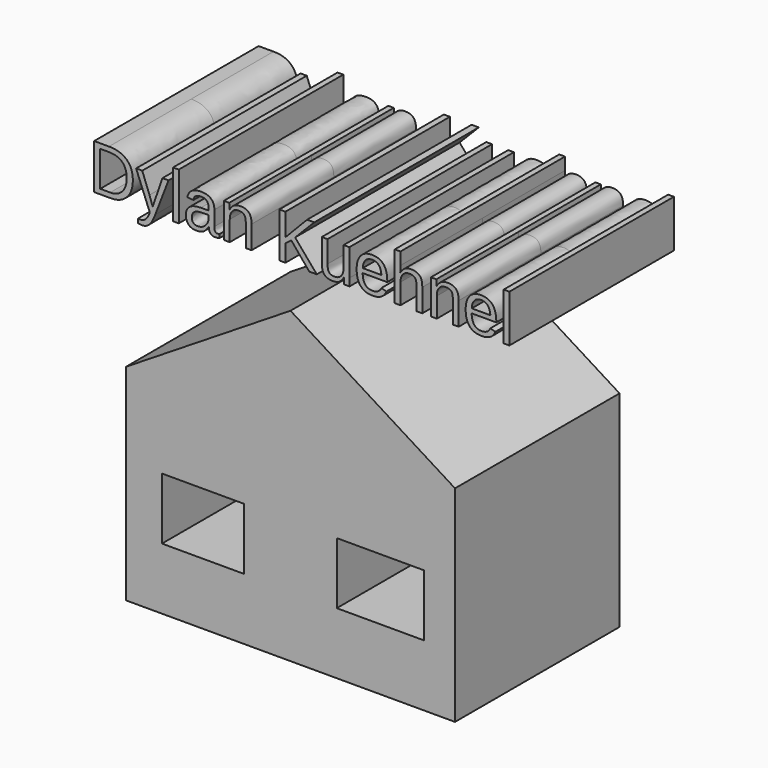
from build123d import *

# Parameters (mm, degrees)
F0_W         = 2438.4
F0_H         = 1828.8
F0_W_2       = 2590.8
F0_TEXT_SIZE = 1936.8767738342
F1_DEPTH     = 3048


# Not quite as in the source:
# - Text() gives the source's letters only with a copy of the font that has no kerning and outlines rounded to 1/6400 em; it was checked with that copy


with BuildPart() as f1:
    # F0 (on Front) → F1 (new body, symmetric)
    with BuildSketch(Plane.XZ):
        Polygon((4876.8, 0), (0, 0), (-4876.8, 0), (-4876.8, -6096), (-457.2, -6096), (-457.2, -3962.4), (457.2, -3962.4), (457.2, -6096), (4876.8, -6096), align=None)
        with Locations((-2590.8, -3352.8)):
            Rectangle(F0_W, F0_H, mode=Mode.SUBTRACT)
        with Locations((2667, -3352.8)):
            Rectangle(F0_W_2, F0_H, mode=Mode.SUBTRACT)
        Polygon((-4876.8, 0), (0, 0), (0, 3048), align=None)
        Polygon((0, 3048), (0, 0), (4876.8, 0), align=None)
        Polygon((-457.2, -3962.4), (-457.2, -6096), (0, -6096), (457.2, -6096), (457.2, -3962.4), align=None)
        with Locations((-5980.0128936768, 4251.2354850769)):
            Text('Dylan Kuehnel', F0_TEXT_SIZE, font='Arimo', text_align=(TextAlign.LEFT, TextAlign.BOTTOM))
    extrude(amount=F1_DEPTH, both=True)


solid = f1.part
